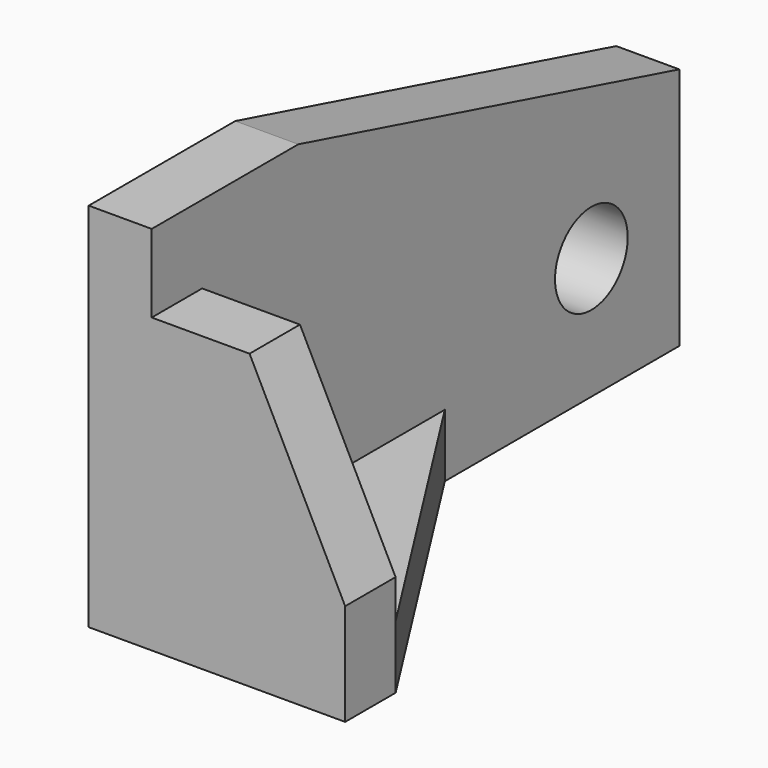
from build123d import *

# Parameters (mm, degrees)
F0_R     = 7.874
F1_DEPTH = 10.922
F0_W     = 52.578
F0_H     = 10.922
F2_DEPTH = 44.45
F3_SIZE2 = 33.1422148526
F3_SIZE  = 16.5711074262
F4_SIZE2 = 52.567648
F4_SIZE  = 33.52799


# Not quite as in the source:
# - a fillet or chamfer is up to 0.001 mm smaller than in the source, because OpenCascade refuses the exact size


with BuildPart() as f1:
    # F0 (on Right) → F1 (new body)
    with BuildSketch(Plane.YZ):
        Polygon((-41.4015134737, 34.2036390094), (-73.1515134737, 34.2036390094), (-73.1515134737, 20.6804594447), (-62.2295134737, 20.6804594447), (-62.2295134737, -19.1975405553), (-9.6515134737, -19.1975405553), (-9.6515134737, -30.1195405553), (41.1484865263, -30.1195405553), (41.1484865263, 12.0844331742), align=None)
        with Locations((22.0984865263, -9.0175536905)):
            Circle(F0_R, mode=Mode.SUBTRACT)
    extrude(amount=F1_DEPTH)

    # F0 (on Right) → F2 (join)
    with BuildSketch(Plane.YZ):
        with Locations((-35.9405134737, -24.6585405553)):
            Rectangle(F0_W, F0_H)
        Polygon((-62.2295134737, 20.6804594447), (-73.1515134737, 20.6804594447), (-73.1515134737, -30.1195405553), (-62.2295134737, -30.1195405553), (-62.2295134737, -19.1975405553), align=None)
    extrude(amount=F2_DEPTH)

    # F3
    f3_edges = [f1.edges().sort_by_distance(p)[0] for p in [
        (44.45, -67.690513, 20.680459),
    ]]
    f3_side = f1.faces().sort_by_distance((27.686, -67.690513, 20.680459))[0]
    chamfer(f3_edges, length=F3_SIZE, length2=F3_SIZE2, reference=f3_side)

    # F4 (size 33.528 and 52.5676582111 in the source; OpenCascade refuses exactly that, so slightly less here)
    f4_edges = [f1.edges().sort_by_distance(p)[0] for p in [
        (44.45, -9.651513, -24.658541),
    ]]
    f4_side = f1.faces().sort_by_distance((27.686, -9.651513, -24.658541))[0]
    chamfer(f4_edges, length=F4_SIZE, length2=F4_SIZE2, reference=f4_side)


solid = f1.part
